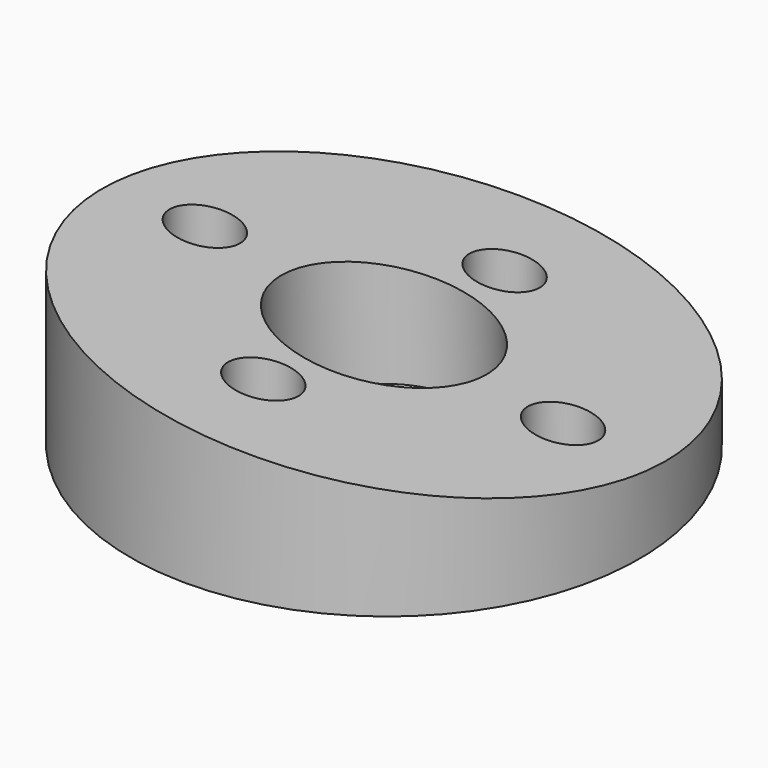
from build123d import *

# Parameters (mm, degrees)
F0_R     = 14
F0_R_2   = 1.75
F0_R_3   = 5.1
F1_DEPTH = 10
F6_DEPTH = 40


with BuildPart() as f1:
    # F0 (on Top) → F1 (new body)
    with BuildSketch(Plane.XY):
        Circle(F0_R)
        with Locations((0, -8)):
            Circle(F0_R_2, mode=Mode.SUBTRACT)
        with Locations((-9.5, 0)):
            Circle(F0_R_2, mode=Mode.SUBTRACT)
        Circle(F0_R_3, mode=Mode.SUBTRACT)
        with Locations((9.5, 0)):
            Circle(F0_R_2, mode=Mode.SUBTRACT)
        with Locations((0, 8)):
            Circle(F0_R_2, mode=Mode.SUBTRACT)
    extrude(amount=F1_DEPTH)

    # F5 (on face) → F6 (intersect)
    with BuildSketch(Plane(origin=(17.6564226245, -17.6564226245, -1.2253490154), x_dir=(0.7045622489, 0.7079556371, -0.0488963521), z_dir=(0.706256905, -0.706256905, -0.0490139606))):
        Polygon((-42.1593469174, 12.1424701935), (-41.5246425416, -0.8069908946), (14.9219552549, 1.9596804268), (14.7750896798, 4.9560833541), align=None)
        Polygon((14.7750896798, 4.9560833541), (14.9219552549, 1.9596804268), (31.9154007009, 2.7925964926), align=None)
    extrude(amount=-F6_DEPTH, mode=Mode.INTERSECT)


solid = f1.part
